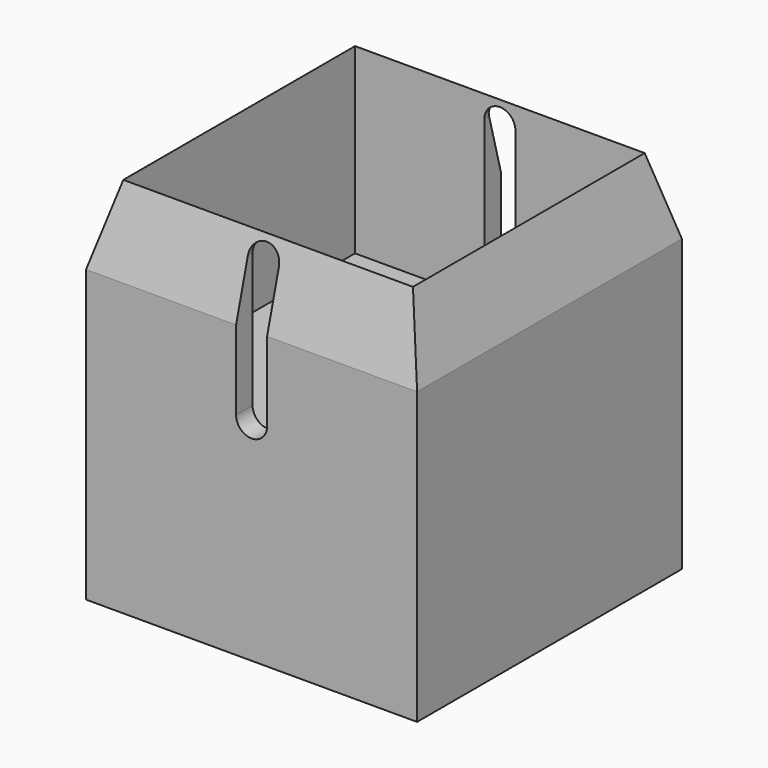
from build123d import *

# Parameters (mm, degrees)
F0_W           = 50.8
F0_H           = 50.8
F1_DEPTH       = 56.45
F2_W           = 44.45
F2_H           = 44.45
F3_DEPTH       = 28
F5_D           = 11
F5_CBORE_D     = 17.25
F5_CBORE_DEPTH = 10
F6_SIZE2       = 11.849251
F6_SIZE        = 3.17499
F8_W           = 4.7625
F8_H           = 20.6375
F9_DEPTH       = 50.801


# Not quite as in the source:
# - a fillet or chamfer is up to 0.001 mm smaller than in the source, because OpenCascade refuses the exact size


with BuildPart() as f1:
    # F0 (on Top) → F1 (new body)
    with BuildSketch(Plane.XY):
        Rectangle(F0_W, F0_H)
    extrude(amount=F1_DEPTH)

    # F2 (on face) → F3 (cut)
    with BuildSketch(Plane.XY.offset(56.45)):
        Rectangle(F2_W, F2_H)
    extrude(amount=-F3_DEPTH, mode=Mode.SUBTRACT)

    # F5 (through all)
    with Locations(Plane.XY.offset(28.45)):
        with Locations((0, 0)):
            CounterBoreHole(F5_D / 2, F5_CBORE_D / 2, F5_CBORE_DEPTH)

    # F6 (size 3.175 and 11.849261314 in the source; OpenCascade refuses exactly that, so slightly less here)
    f6_edges = [f1.edges().sort_by_distance(p)[0] for p in [
        (0, 25.4, 56.45),
        (25.4, 0, 56.45),
        (0, -25.4, 56.45),
        (-25.4, 0, 56.45),
    ]]
    f6_side = f1.faces().sort_by_distance((0, -24.68158, 56.45))[0]
    chamfer(f6_edges, length=F6_SIZE, length2=F6_SIZE2, reference=f6_side)

    # F8 (on offset) → F9 (cut, through all)
    with BuildSketch(Plane(origin=(0, 25.4, 0), x_dir=(-1, 0, 0), z_dir=(0, 1, 0))):
        with BuildLine():
            ThreePointArc((-2.38125, 32.41875), (0, 30.0375), (2.38125, 32.41875))
            Line((2.38125, 32.41875), (-2.38125, 32.41875))
        make_face()
        with Locations((0, 42.7375)):
            Rectangle(F8_W, F8_H)
        with BuildLine():
            Line((-2.38125, 53.05625), (2.38125, 53.05625))
            ThreePointArc((2.38125, 53.05625), (0, 55.4375), (-2.38125, 53.05625))
        make_face()
    extrude(amount=-F9_DEPTH, mode=Mode.SUBTRACT)


solid = f1.part
